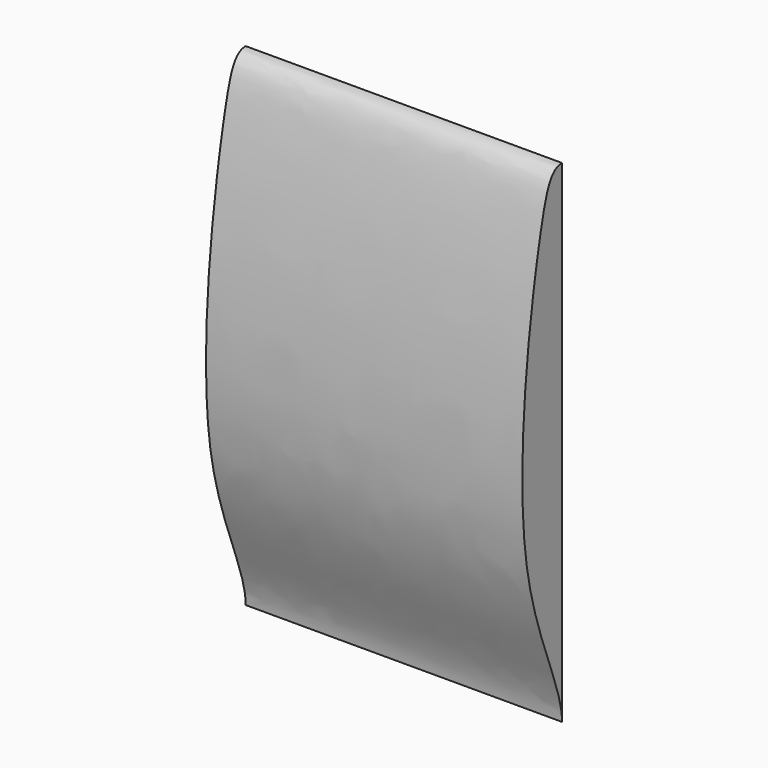
from build123d import *

# Parameters (mm, degrees)
F1_DEPTH       = 457.2
F2_W           = 95.25
F2_H           = 355.6
F3_DEPTH       = 57.15
F4_W           = 57.15
F4_H           = 6.35
F5_DEPTH       = 355.6
F7_D           = 6.35
F7_DEPTH       = 6.35
F7_CSINK_D     = 12.7
F7_CSINK_ANGLE = 90
F7_TIP         = 1.9077324654


with BuildPart() as f1:
    # F0 (on Right) → F1 (new body)
    with BuildSketch(Plane.YZ):
        with BuildLine():
            Line((0, 0), (0, 711.2))
            add(Edge.make_bspline(
                [(0, 711.2), (-20.1591427607, 711.2), (-45.7016939777, 633.1559120736), (-107.7342542848, 213.8871421657), (0, 46.9480343163), (0, 0)],
                knots=[0, 0, 0, 0, 0.1909577513, 0.6605552896, 1, 1, 1, 1], degree=3))
        make_face()
    extrude(amount=F1_DEPTH)

    # F2 (on face) → F3 (join)
    with BuildSketch(Plane(origin=(0, 0, 0), x_dir=(-1, 0, 0), z_dir=(0, 1, 0))):
        with Locations((-228.6, 355.6)):
            Rectangle(F2_W, F2_H)
    extrude(amount=F3_DEPTH)

    # F4 (on face) → F5 (cut)
    with BuildSketch(Plane.XY.offset(533.4)):
        Polygon((269.875, 50.8), (257.175, 50.8), (200.025, 50.8), (187.325, 50.8), (187.325, 0), (269.875, 0), align=None)
        with Locations((228.6, 53.975)):
            Rectangle(F4_W, F4_H)
    extrude(amount=-F5_DEPTH, mode=Mode.SUBTRACT)

    # F7
    with Locations(Plane(origin=(0, 0, 0), x_dir=(-1, 0, 0), z_dir=(0, 1, 0))):
        with Locations((-228.6, 533.4), (-228.6, 488.95), (-228.6, 444.5), (-228.6, 400.05), (-228.6, 355.6), (-228.6, 311.15), (-228.6, 266.7)):
            CounterSinkHole(F7_D / 2, F7_CSINK_D / 2, depth=F7_DEPTH, counter_sink_angle=F7_CSINK_ANGLE)
            with Locations((0, 0, -(F7_DEPTH + F7_TIP / 2))):  # 118° drill point
                Cone(0, F7_D / 2, F7_TIP, mode=Mode.SUBTRACT)


solid = f1.part
